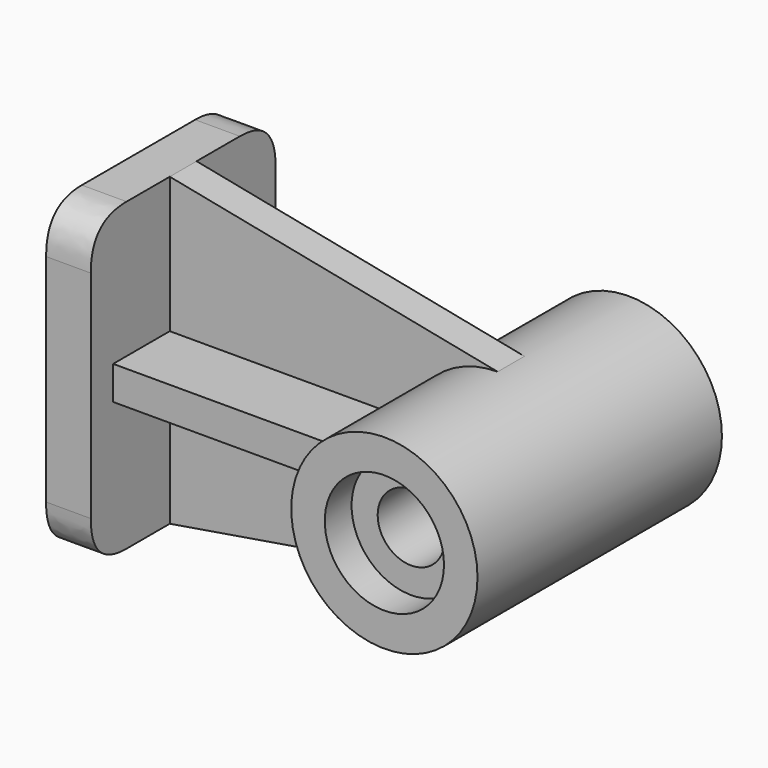
from build123d import *

# Parameters (mm, degrees)
F0_W            = 62
F0_H            = 82
F1_DEPTH        = 12
F2_T1_DEPTH     = 72
F4_R            = 25
F5_DEPTH        = 42.5
F5_DEPTH_BACK   = 39.5
F3_W            = 19
F3_H            = 9
F6_DEPTH        = 88
F8_DEPTH        = 25
F10_DEPTH       = 25
F12_D           = 18
F12_DEPTH       = 90
F12_CBORE_D     = 32
F12_CBORE_DEPTH = 9
F12_TIP         = 5.4077455712


# Not quite as in the source:
# - a fillet or chamfer that OpenCascade refuses, or shapes differently, is made with other operations: its cross-section is extruded or revolved along the edge and cut away or added


with BuildPart() as f1:
    # F0 (on Right) → F1 (new body)
    with BuildSketch(Plane.YZ):
        with Locations((0, 1.4735981822)):
            Rectangle(F0_W, F0_H)
    extrude(amount=F1_DEPTH)

    # F2: fillet of radius 12 on 4 edges, made by hand

    # F2_s2 → F2_t1 (cut)
    with BuildSketch(Plane.YZ.offset(-30)):
        with BuildLine():
            add(Edge.make_bspline(
                [(-19, 42.4735981822), (-31, 42.4735981822), (-31, 30.4735981822)],
                knots=[0, 0, 0, 1, 1, 1], degree=2, weights=[1, 1, 1]))
            Line((-31, 30.4735981822), (-31, 42.4735981822))
            Line((-31, 42.4735981822), (-19, 42.4735981822))
        make_face()
        with BuildLine():
            add(Edge.make_bspline(
                [(31, 30.4735981822), (31, 42.4735981822), (19, 42.4735981822)],
                knots=[0, 0, 0, 1, 1, 1], degree=2, weights=[1, 1, 1]))
            Line((19, 42.4735981822), (31, 42.4735981822))
            Line((31, 42.4735981822), (31, 30.4735981822))
        make_face()
        with BuildLine():
            add(Edge.make_bspline(
                [(-31, -27.5264018178), (-31, -39.5264018178), (-19, -39.5264018178)],
                knots=[0, 0, 0, 1, 1, 1], degree=2, weights=[1, 1, 1]))
            Line((-19, -39.5264018178), (-31, -39.5264018178))
            Line((-31, -39.5264018178), (-31, -27.5264018178))
        make_face()
        with BuildLine():
            add(Edge.make_bspline(
                [(31, -27.5264018178), (31, -39.5264018178), (19, -39.5264018178)],
                knots=[0, 0, 0, 1, 1, 1], degree=2, weights=[1, 1, 1]))
            Line((19, -39.5264018178), (31, -39.5264018178))
            Line((31, -39.5264018178), (31, -27.5264018178))
        make_face()
    extrude(amount=F2_T1_DEPTH, mode=Mode.SUBTRACT)



with BuildPart() as f5:
    # F4 (on Front) → F5 (new body, two sides)
    with BuildSketch(Plane.XZ) as f5_sk:
        with Locations((100, 0)):
            Circle(F4_R)
    extrude(amount=F5_DEPTH)
    extrude(f5_sk.sketch, amount=-F5_DEPTH_BACK)


with BuildPart() as f1_1:
    add(f1.part)

    add(f5.part)  # F6 merges F5
    # F3 (on face) → F6 (join)
    with BuildSketch(Plane.YZ.offset(12)):
        Polygon((4.5, 5.9735981822), (4.5, 42.4735981822), (-4.5, 42.4735981822), (-4.5, 5.9735981822), (-4.5, -3.0264018178), (-4.5, -39.5264018178), (4.5, -39.5264018178), (4.5, -3.0264018178), (23.5, -3.0264018178), (23.5, 5.9735981822), align=None)
        with Locations((-14, 1.4735981822)):
            Rectangle(F3_W, F3_H)
    extrude(amount=F6_DEPTH)

    # F7 (on face) → F8 (cut)
    with BuildSketch(Plane.XZ.offset(4.5)):
        Polygon((100, 42.4735981822), (12, 42.4735981822), (100, 25), align=None)
    extrude(amount=-F8_DEPTH, mode=Mode.SUBTRACT)

    # F9 (on face) → F10 (cut)
    with BuildSketch(Plane.XZ.offset(4.5)):
        Polygon((100, -39.5264018178), (100, -25), (12, -39.5264018178), align=None)
    extrude(amount=-F10_DEPTH, mode=Mode.SUBTRACT)

    # F12
    with Locations(Plane.XZ.offset(42.5)):
        with Locations((100, 0)):
            CounterBoreHole(F12_D / 2, F12_CBORE_D / 2, F12_CBORE_DEPTH, depth=F12_DEPTH)
            with Locations((0, 0, -(F12_DEPTH + F12_TIP / 2))):  # 118° drill point
                Cone(0, F12_D / 2, F12_TIP, mode=Mode.SUBTRACT)


solid = f1_1.part
